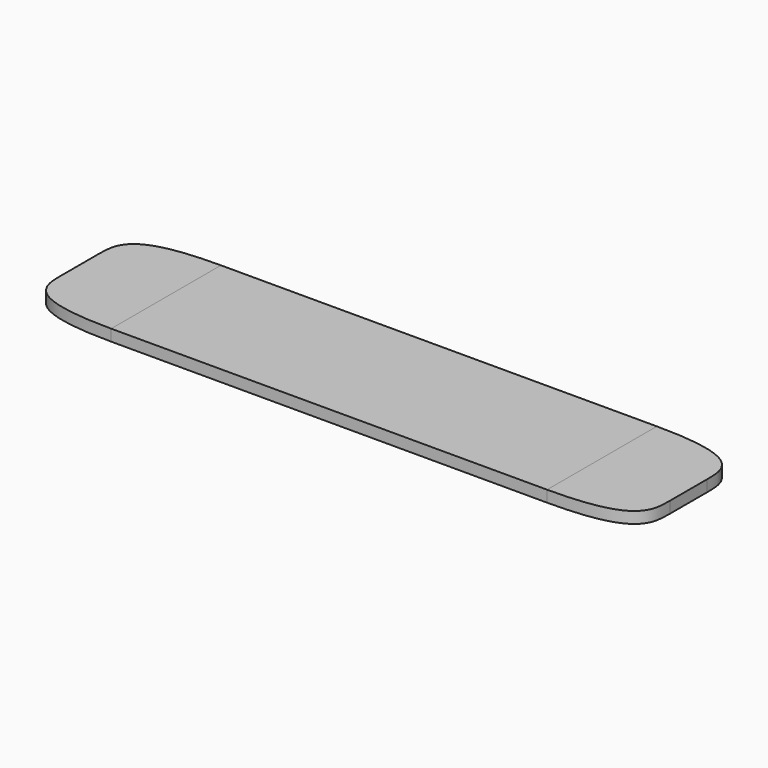
from build123d import *

# Parameters (mm, degrees)
F1_DEPTH = 19.05
F2_DEPTH = 19.05


# Not quite as in the source:
# - ends of sketch curves that miss each other by under 0.0002 mm in the source are joined


with BuildPart() as f1:
    # F0 (on Top) → F1 (new body)
    with BuildSketch(Plane.XY):
        Polygon((-362.6891076565, 114.2999976873), (-362.6891076565, -114.3000023127), (363.7220774023, -114.3), (363.7220774023, 114.3), align=None)
    extrude(amount=F1_DEPTH)


with BuildPart() as f2:
    # F0 (on Top) → F2 (new body)
    with BuildSketch(Plane.XY):
        with BuildLine():
            Line((363.7220774023, 114.3), (363.7220774023, -114.3))
            add(Edge.make_bspline(
                [(508, -38.1), (508, -75.5596795078), (508, -114.3), (363.7220774023, -114.3)],
                knots=[0.6273362794, 0.6273362794, 0.6273362794, 0.6273362794, 1, 1, 1, 1], degree=3))
            Line((508, -38.1), (508, 38.1))
            add(Edge.make_bspline(
                [(363.7220774023, 114.3), (508, 114.3), (508, 75.5596795078), (508, 38.1)],
                knots=[0, 0, 0, 0, 0.3726637206, 0.3726637206, 0.3726637206, 0.3726637206], degree=3))
        make_face()
    extrude(amount=F2_DEPTH)


with BuildPart() as f2b:
    # F0 (on Top) → F2, piece 2 (new body)
    with BuildSketch(Plane.XY):
        with BuildLine():
            add(Edge.make_bspline(
                [(-362.6891076565, -114.3000023127), (-506.9670302542, -114.3000023127), (-506.9670302542, -75.5596818205), (-506.9670302542, -38.1000023127)],
                knots=[0, 0, 0, 0, 0.3726637206, 0.3726637206, 0.3726637206, 0.3726637206], degree=3))
            Line((-362.6891076565, -114.3000023127), (-362.6891076565, 114.2999976873))
            add(Edge.make_bspline(
                [(-506.9670302542, 38.0999976873), (-506.9670302542, 75.5596771952), (-506.9670302542, 114.2999976873), (-362.6891076565, 114.2999976873)],
                knots=[0.6273362794, 0.6273362794, 0.6273362794, 0.6273362794, 1, 1, 1, 1], degree=3))
            Line((-506.9670302542, 38.0999976873), (-506.9670302542, -38.1000023127))
        make_face()
    extrude(amount=F2_DEPTH)


solid = Compound([f1.part, f2.part, f2b.part])
